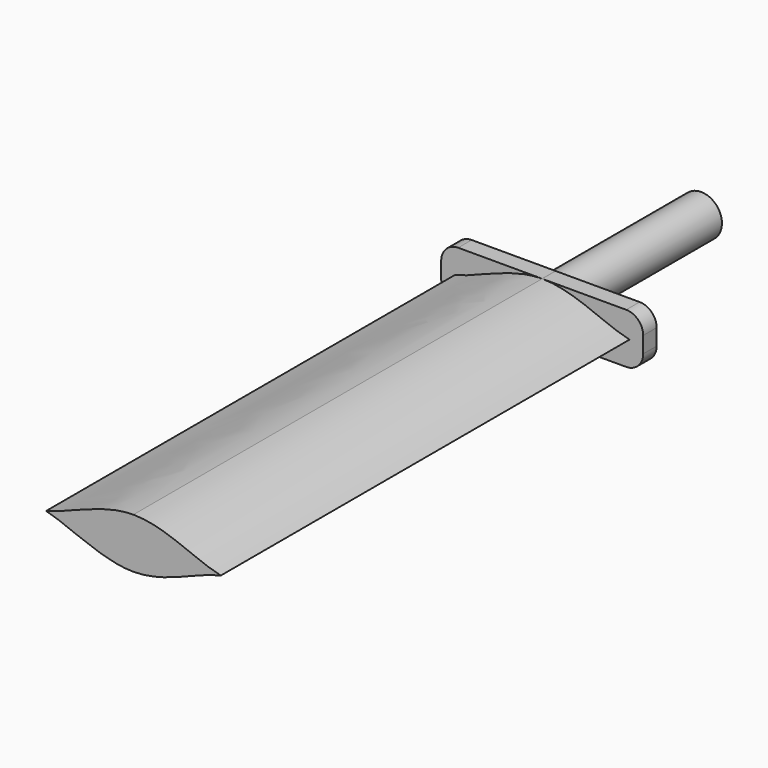
from build123d import *

# Parameters (mm, degrees)
F1_DEPTH = 12.53708
F2_DEPTH = 148.17746
F3_DEPTH = 381


# Not quite as in the source:
# - ends of sketch curves that miss each other by under 0.0002 mm in the source are joined
# - a feature names something its author has since deleted; it is built from what else it names


with BuildPart() as f1:
    # F0 (on Front) → F1 (new body)
    with BuildSketch(Plane.XZ):
        with BuildLine():
            Line((-0.0432951165, 18.7523439527), (-62.6219127655, 18.7523439527))
            ThreePointArc((-62.6219127655, 18.7523439527), (-71.6021688866, 15.0326000737), (-75.3219127655, 6.0523439527))
            Line((-75.3219127655, 6.0523439527), (-75.3219127655, 0))
            Line((-75.3219127655, 0), (-65.1619127655, 0))
            add(Edge.make_bspline(
                [(-65.1619127655, 0), (-48.671609143, 3.823998258), (-23.9979293543, 18.7523570586), (-0.0432951165, 18.7523439527)],
                knots=[0, 0, 0, 0, 0.499698946, 0.499698946, 0.499698946, 0.499698946], degree=3))
        make_face()
        with BuildLine():
            add(Edge.make_bspline(
                [(-0.0432951165, 18.7523602083), (-0.0288631494, 18.7523602102), (23.9542012968, 18.7433586286), (47.2111099504, 3.7542823594), (65.1619127655, 0)],
                knots=[0.499698946, 0.499698946, 0.499698946, 0.499698946, 0.5, 1, 1, 1, 1], degree=3))
            add(Edge.make_bspline(
                [(-65.1619127655, 0), (-48.671609143, 3.823998258), (-23.9979293543, 18.7523570586), (-0.0432951165, 18.7523602083)],
                knots=[0, 0, 0, 0, 0.499698946, 0.499698946, 0.499698946, 0.499698946], degree=3))
            Line((-65.1619127655, 0), (-15.5171778125, 0))
            ThreePointArc((-15.5171778125, 0), (0, 15.5171778125), (15.5171778125, 0))
            Line((15.5171778125, 0), (65.1619127655, 0))
        make_face()
        with BuildLine():
            Line((62.6219127655, 18.7523439527), (-0.0432951165, 18.7523439527))
            add(Edge.make_bspline(
                [(-0.0432951165, 18.7523439527), (-0.0288631494, 18.7523602102), (23.9542012968, 18.7433586286), (47.2111099504, 3.7542823594), (65.1619127655, 0)],
                knots=[0.499698946, 0.499698946, 0.499698946, 0.499698946, 0.5, 1, 1, 1, 1], degree=3))
            Line((65.1619127655, 0), (75.3219127655, 0))
            Line((75.3219127655, 0), (75.3219127655, 6.0523439527))
            ThreePointArc((75.3219127655, 6.0523439527), (71.6021688866, 15.0326000737), (62.6219127655, 18.7523439527))
        make_face()
        with BuildLine():
            add(Edge.make_bspline(
                [(-65.1619127655, 0), (-48.671609143, -3.823998258), (-23.9979293543, -18.7523570586), (-0.0432951165, -18.7523602083)],
                knots=[0, 0, 0, 0, 0.499698946, 0.499698946, 0.499698946, 0.499698946], degree=3))
            Line((-65.1619127655, 0), (-75.3219127655, 0))
            Line((-75.3219127655, 0), (-75.3219127655, -6.0523439527))
            ThreePointArc((-75.3219127655, -6.0523439527), (-71.6021688866, -15.0326000737), (-62.6219127655, -18.7523439527))
            Line((-62.6219127655, -18.7523439527), (-0.0432951165, -18.7523602083))
        make_face()
        with BuildLine():
            Line((-15.5171778125, 0), (-65.1619127655, 0))
            add(Edge.make_bspline(
                [(-65.1619127655, 0), (-48.671609143, -3.823998258), (-23.9979293543, -18.7523570586), (-0.0432951165, -18.7523602083)],
                knots=[0, 0, 0, 0, 0.499698946, 0.499698946, 0.499698946, 0.499698946], degree=3))
            add(Edge.make_bspline(
                [(-0.0432951165, -18.7523602083), (-0.0288631494, -18.7523602102), (23.9542012968, -18.7433586286), (47.2111099504, -3.7542823594), (65.1619127655, 0)],
                knots=[0.499698946, 0.499698946, 0.499698946, 0.499698946, 0.5, 1, 1, 1, 1], degree=3))
            Line((65.1619127655, 0), (15.5171778125, 0))
            ThreePointArc((15.5171778125, 0), (0, -15.5171778125), (-15.5171778125, 0))
        make_face()
        with BuildLine():
            Line((75.3219127655, 0), (65.1619127655, 0))
            add(Edge.make_bspline(
                [(-0.0432951165, -18.7523602083), (-0.0288631494, -18.7523602102), (23.9542012968, -18.7433586286), (47.2111099504, -3.7542823594), (65.1619127655, 0)],
                knots=[0.499698946, 0.499698946, 0.499698946, 0.499698946, 0.5, 1, 1, 1, 1], degree=3))
            Line((-0.0432951165, -18.7523602083), (62.6219127655, -18.7523439527))
            ThreePointArc((62.6219127655, -18.7523439527), (71.6021688866, -15.0326000737), (75.3219127655, -6.0523439527))
            Line((75.3219127655, -6.0523439527), (75.3219127655, 0))
        make_face()
        with BuildLine():
            ThreePointArc((15.5171778125, 0), (0, 15.5171778125), (-15.5171778125, 0))
            ThreePointArc((-15.5171778125, 0), (0, -15.5171778125), (15.5171778125, 0))
        make_face()
    extrude(amount=-F1_DEPTH)

    # F0 (on Front) → F2 (join)
    with BuildSketch(Plane.XZ):
        with BuildLine():
            ThreePointArc((15.5171778125, 0), (0, 15.5171778125), (-15.5171778125, 0))
            ThreePointArc((-15.5171778125, 0), (0, -15.5171778125), (15.5171778125, 0))
        make_face()
    extrude(amount=-F2_DEPTH)

    # F0 (on Front) → F3 (join)
    with BuildSketch(Plane.XZ):
        with BuildLine():
            add(Edge.make_bspline(
                [(-0.0432951165, 18.7523602083), (-0.0288631494, 18.7523602102), (23.9542012968, 18.7433586286), (47.2111099504, 3.7542823594), (65.1619127655, 0)],
                knots=[0.499698946, 0.499698946, 0.499698946, 0.499698946, 0.5, 1, 1, 1, 1], degree=3))
            add(Edge.make_bspline(
                [(-65.1619127655, 0), (-48.671609143, 3.823998258), (-23.9979293543, 18.7523570586), (-0.0432951165, 18.7523602083)],
                knots=[0, 0, 0, 0, 0.499698946, 0.499698946, 0.499698946, 0.499698946], degree=3))
            Line((-65.1619127655, 0), (-15.5171778125, 0))
            ThreePointArc((-15.5171778125, 0), (0, 15.5171778125), (15.5171778125, 0))
            Line((15.5171778125, 0), (65.1619127655, 0))
        make_face()
        with BuildLine():
            Line((-15.5171778125, 0), (-65.1619127655, 0))
            add(Edge.make_bspline(
                [(-65.1619127655, 0), (-48.671609143, -3.823998258), (-23.9979293543, -18.7523570586), (-0.0432951165, -18.7523602083)],
                knots=[0, 0, 0, 0, 0.499698946, 0.499698946, 0.499698946, 0.499698946], degree=3))
            add(Edge.make_bspline(
                [(-0.0432951165, -18.7523602083), (-0.0288631494, -18.7523602102), (23.9542012968, -18.7433586286), (47.2111099504, -3.7542823594), (65.1619127655, 0)],
                knots=[0.499698946, 0.499698946, 0.499698946, 0.499698946, 0.5, 1, 1, 1, 1], degree=3))
            Line((65.1619127655, 0), (15.5171778125, 0))
            ThreePointArc((15.5171778125, 0), (0, -15.5171778125), (-15.5171778125, 0))
        make_face()
        with BuildLine():
            ThreePointArc((15.5171778125, 0), (0, 15.5171778125), (-15.5171778125, 0))
            ThreePointArc((-15.5171778125, 0), (0, -15.5171778125), (15.5171778125, 0))
        make_face()
    extrude(amount=F3_DEPTH)


solid = f1.part
